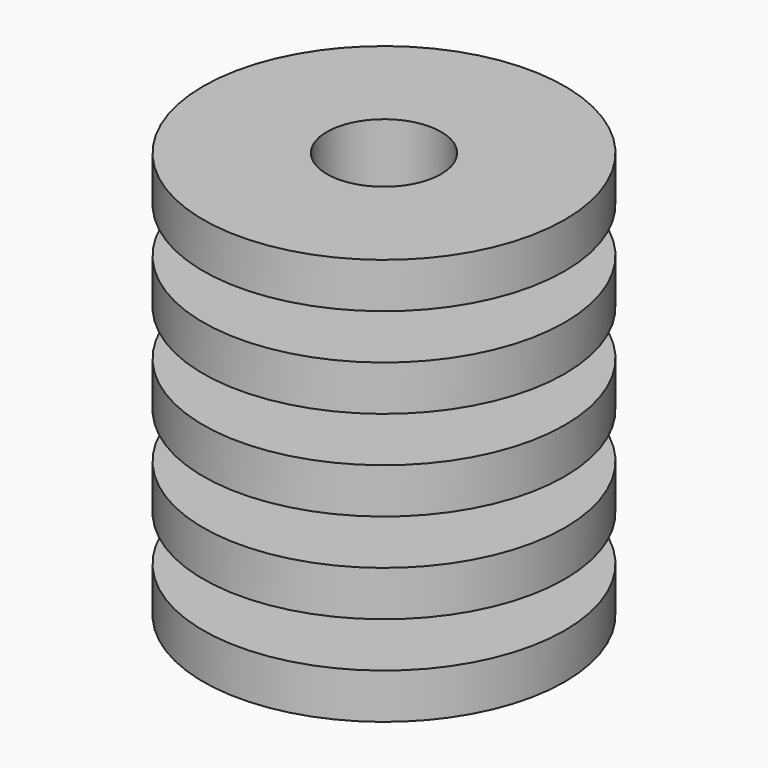
from build123d import *

# Parameters (mm, degrees)
F3_R     = 18.2754285366
F4_DEPTH = 251
F5_R     = 16.060733565
F6_DEPTH = 127.001


# Not quite as in the source:
# - an extrude ends at something that could not be found from the text; its depth is read off the source's solid


with BuildPart() as f1:
    # F0 (on Front) → F1 (revolve)
    with BuildSketch(Plane.XZ):
        Polygon((0, 127), (0, 0), (19.05, 0), (19.05, 12.7), (50.8, 12.7), (50.8, 25.4), (19.05, 25.4), (19.05, 38.1), (50.8, 38.1), (50.8, 50.8), (19.05, 50.8), (19.05, 63.5), (50.8, 63.5), (50.8, 76.2), (19.05, 76.2), (19.05, 88.9), (50.8, 88.9), (50.8, 101.6), (19.05, 101.6), (19.05, 114.3), (50.8, 114.3), (50.8, 127), align=None)
    revolve(axis=Axis((0, 0, 63.5), (0, 0, 1)))

    # F3 (on face) → F4 (cut, through all)
    with BuildSketch(Plane.XY.offset(127)):
        Circle(F3_R)
    extrude(amount=F4_DEPTH, mode=Mode.SUBTRACT)

    # F5 (on face) → F6 (cut, through all)
    with BuildSketch(Plane.XY.offset(127)):
        Circle(F5_R)
    extrude(amount=-F6_DEPTH, mode=Mode.SUBTRACT)


solid = f1.part
